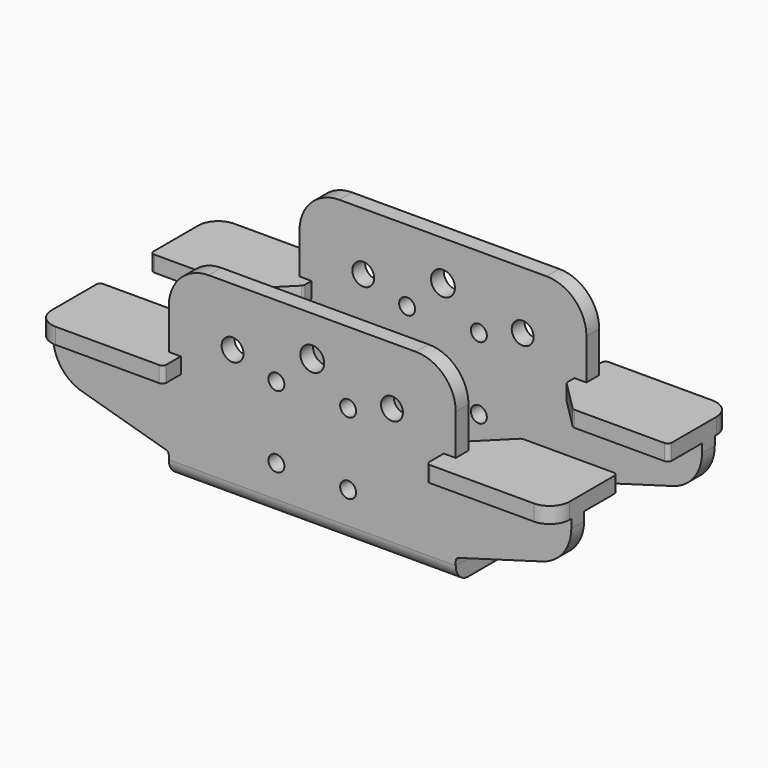
from build123d import *

# Parameters (mm, degrees)
F0_R          = 2
F0_R_2        = 2.75
F0_R_3        = 3
F1_DEPTH      = 4
F2_DEPTH      = 14.5
F2_DEPTH_BACK = 5.5
F3_R          = 5
F4_R          = 1
F5_SIZE       = 8
F6_R          = 1
F9_W          = 72
F9_H          = 45
F9_W_2        = 8.2
F9_H_2        = 4.2
F9_R          = 17.5
F10_DEPTH     = 4
F11_R         = 3.99999
F12_DEPTH     = 1
F13_DEPTH     = 1


# Not quite as in the source:
# - a fillet or chamfer is up to 0.001 mm smaller than in the source, because OpenCascade refuses the exact size


with BuildPart() as f1:
    # F0 (on Front) → F1 (new body)
    with BuildSketch(Plane.XZ):
        with BuildLine():
            Line((-36, 5), (-36, 3))
            Line((-36, 3), (36, 3))
            Line((36, 3), (36, 5))
            Line((36, 5), (36, 23.8))
            Line((36, 23.8), (33, 23.8))
            Line((33, 23.8), (33, 27.8))
            Line((33, 27.8), (36, 27.8))
            Line((36, 27.8), (36, 38))
            ThreePointArc((36, 38), (33.0710678119, 45.0710678119), (26, 48))
            Line((26, 48), (-26, 48))
            ThreePointArc((-26, 48), (-33.0710678119, 45.0710678119), (-36, 38))
            Line((-36, 38), (-36, 27.8))
            Line((-36, 27.8), (-33, 27.8))
            Line((-33, 27.8), (-33, 23.8))
            Line((-33, 23.8), (-36, 23.8))
            Line((-36, 23.8), (-36, 5))
        make_face()
        with Locations((-9, 12)):
            Circle(F0_R, mode=Mode.SUBTRACT)
        with Locations((9, 12)):
            Circle(F0_R, mode=Mode.SUBTRACT)
        with Locations((-20, 33.5)):
            Circle(F0_R_2, mode=Mode.SUBTRACT)
        with Locations((-9, 30)):
            Circle(F0_R, mode=Mode.SUBTRACT)
        with Locations((9, 30)):
            Circle(F0_R, mode=Mode.SUBTRACT)
        with Locations((20, 33.5)):
            Circle(F0_R_2, mode=Mode.SUBTRACT)
        with Locations((0, 38)):
            Circle(F0_R_3, mode=Mode.SUBTRACT)
        with BuildLine():
            Line((36, 23.8), (36, 5))
            ThreePointArc((36, 5), (36.2012712878, 5.6016913198), (36.7240648886, 5.961176266))
            Line((36.7240648886, 5.961176266), (57.7593511139, 12))
            ThreePointArc((57.7593511139, 12), (62.987287122, 15.594849462), (65, 21.6117626599))
            Line((65, 21.6117626599), (65, 23.8))
            Line((65, 23.8), (36, 23.8))
        make_face()
        with BuildLine():
            ThreePointArc((-36.7240648886, 5.961176266), (-36.2012712878, 5.6016913198), (-36, 5))
            Line((-36, 5), (-36, 23.8))
            Line((-36, 23.8), (-65, 23.8))
            Line((-65, 23.8), (-65, 21.6117626599))
            ThreePointArc((-65, 21.6117626599), (-62.987287122, 15.594849462), (-57.7593511139, 12))
            Line((-57.7593511139, 12), (-36.7240648886, 5.961176266))
        make_face()
    extrude(amount=F1_DEPTH)

    # F0 (on Front) → F2 (join, two sides)
    with BuildSketch(Plane.XZ) as f2_sk:
        Polygon((33, 23.8), (36, 23.8), (65, 23.8), (65, 27.8), (36, 27.8), (33, 27.8), align=None)
        Polygon((-65, 23.8), (-36, 23.8), (-33, 23.8), (-33, 27.8), (-36, 27.8), (-65, 27.8), align=None)
    extrude(amount=F2_DEPTH)
    extrude(f2_sk.sketch, amount=-F2_DEPTH_BACK)

    # F3
    f3_edges = [f1.edges().sort_by_distance(p)[0] for p in [
        (-65, 5.5, 25.8),
        (65, 5.5, 25.8),
    ]]
    fillet(f3_edges, radius=F3_R)

    # F4
    f4_edges = [f1.edges().sort_by_distance(p)[0] for p in [
        (-65, -14.5, 25.8),
        (-33, 5.5, 25.8),
        (65, -14.5, 25.8),
        (33, 5.5, 25.8),
    ]]
    fillet(f4_edges, radius=F4_R)

    # F5
    f5_edges = [f1.edges().sort_by_distance(p)[0] for p in [
        (33, -14.5, 25.8),
        (-33, -14.5, 25.8),
    ]]
    chamfer(f5_edges, length=F5_SIZE)

    # F6
    f6_edges = [f1.edges().sort_by_distance(p)[0] for p in [
        (41, -14.5, 25.8),
        (33, -6.5, 25.8),
        (-33, -6.5, 25.8),
        (-41, -14.5, 25.8),
    ]]
    fillet(f6_edges, radius=F6_R)


with BuildPart() as f1_1:
    # F7: moved
    add(f1.part.moved(Location((0, 22.5, 0))))


with BuildPart() as f8_1:
    # F8: instance of F1
    add(f1_1.part.mirror(Plane.XZ))

    # F13 (cut): a face of the model
    f13_faces = [f8_1.faces().sort_by_distance(p)[0] for p in [
        (0, -20.5, 3),
    ]]
    extrude(f13_faces, amount=-F13_DEPTH, mode=Mode.SUBTRACT)


with BuildPart() as f10:
    # F9 (on Top) → F10 (new body)
    with BuildSketch(Plane.XY):
        Rectangle(F9_W, F9_H)
        with Locations((-25.65, 0)):
            Rectangle(F9_W_2, F9_H_2, mode=Mode.SUBTRACT)
        Circle(F9_R, mode=Mode.SUBTRACT)
        with Locations((25.65, 0)):
            Rectangle(F9_W_2, F9_H_2, mode=Mode.SUBTRACT)
    extrude(amount=F10_DEPTH)

    # F11 (radius 4 in the source; OpenCascade refuses exactly that, so slightly less here)
    f11_edges = [f10.edges().sort_by_distance(p)[0] for p in [
        (0, 22.5, 0),
        (0, -22.5, 0),
    ]]
    fillet(f11_edges, radius=F11_R)


with BuildPart() as f1_2:
    add(f1_1.part)

    # F12 (cut): a face of the model
    f12_faces = [f1_2.faces().sort_by_distance(p)[0] for p in [
        (0, 20.5, 3),
    ]]
    extrude(f12_faces, amount=-F12_DEPTH, mode=Mode.SUBTRACT)


solid = Compound([f8_1.part, f10.part, f1_2.part])
